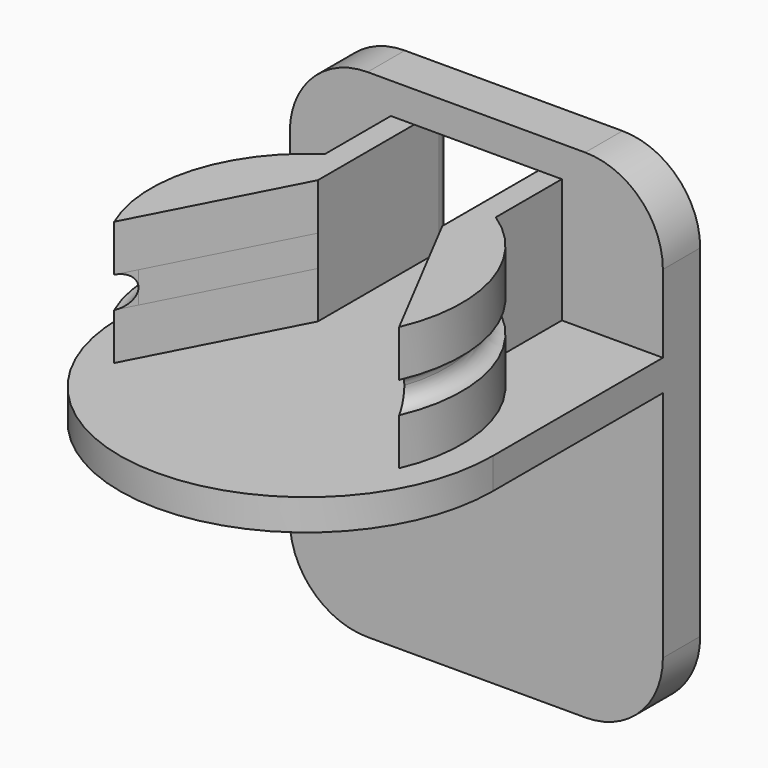
from build123d import *

# Parameters (mm, degrees)
F1_DEPTH     = 2
F3_DEPTH     = 3
F5_DEPTH     = 2
F7_DEPTH     = 3
F8_T4_ANGLE  = 102.3969146675
F8_T10_ANGLE = 102.3969146675
F8_T16_ANGLE = 102.3969146675
F8_T22_ANGLE = 102.3969146675
F8_T26_ANGLE = 121.7069479791
F8_T28_ANGLE = 121.7069479791
F8_T30_ANGLE = 121.7069479791
F8_T32_ANGLE = 121.7069479791
F9_W         = 24
F9_H         = 22.6653645039
F10_DEPTH    = 10
F11_W        = 24
F11_H        = 32
F11_W_2      = 8
F11_H_2      = 8
F12_DEPTH    = 3
F13_R        = 1
F14_R        = 5
F15_W        = 24
F15_H        = 13.6653645039
F16_DEPTH    = 2


# Not quite as in the source:
# - a fillet or chamfer that OpenCascade refuses, or shapes differently, is made with other operations: its cross-section is extruded or revolved along the edge and cut away or added


with BuildPart() as f1:
    # F0 (on Top) → F1 (new body)
    with BuildSketch(Plane.XY):
        with BuildLine():
            ThreePointArc((5.5, 1.5), (0, 24.1653645039), (-5.5, 1.5))
            Line((-5.5, 1.5), (-5.5, -1.5))
            ThreePointArc((-5.5, -1.5), (0, -24.1653645039), (5.5, -1.5))
            Line((5.5, -1.5), (5.5, 1.5))
        make_face()
    extrude(amount=F1_DEPTH)

    # F2 (on face) → F3 (join)
    with BuildSketch(Plane.XY.offset(2)):
        with BuildLine():
            Line((9.7844830762, 19.1125863177), (8.6602540378, 17.1653645039))
            ThreePointArc((8.6602540378, 17.1653645039), (9.4991255677, 9.0402063559), (4, 3.0002131139))
            Line((4, 3.0002131139), (4, -6.2432010007))
            Line((4, -6.2432010007), (9.1651513899, -16.1653645039))
            ThreePointArc((9.1651513899, -16.1653645039), (9.5868378212, -9.3206253964), (5.5, -3.8137179596))
            Line((5.5, -3.8137179596), (5.5, 1.5))
            ThreePointArc((5.5, 1.5), (11.6599594736, 9.3289327537), (9.7844830762, 19.1125863177))
        make_face()
        with BuildLine():
            ThreePointArc((-4, 3.0002131139), (-9.4991255677, 9.0402063559), (-8.6602540378, 17.1653645039))
            Line((-8.6602540378, 17.1653645039), (-9.7844830762, 19.1125863177))
            ThreePointArc((-9.7844830762, 19.1125863177), (-11.6599594736, 9.3289327537), (-5.5, 1.5))
            Line((-5.5, 1.5), (-5.5, -3.8137179596))
            ThreePointArc((-5.5, -3.8137179596), (-9.5868378212, -9.3206253964), (-9.1651513899, -16.1653645039))
            Line((-9.1651513899, -16.1653645039), (-4, -6.2432010007))
            Line((-4, -6.2432010007), (-4, 3.0002131139))
        make_face()
    extrude(amount=F3_DEPTH)

    # F4 (on face) → F5 (join)
    with BuildSketch(Plane.XY.offset(5)):
        with BuildLine():
            Line((-8.0717844057, 16.1461052023), (-9.7844830762, 19.1125863177))
            ThreePointArc((-9.7844830762, 19.1125863177), (-11.6599594736, 9.3289327537), (-5.5, 1.5))
            Line((-5.5, 1.5), (-5.5, -5.0414610795))
            ThreePointArc((-5.5, -5.0414610795), (-8.6043935433, -9.5263473097), (-8.5483759414, -14.980549891))
            Line((-8.5483759414, -14.980549891), (-4, -6.2432010007))
            Line((-4, -6.2432010007), (-4, 4.1031067556))
            ThreePointArc((-4, 4.1031067556), (-8.5258693153, 9.2827350759), (-8.0717844057, 16.1461052023))
        make_face()
        with BuildLine():
            ThreePointArc((5.5, 1.5), (11.6599594736, 9.3289327537), (9.7844830762, 19.1125863177))
            Line((9.7844830762, 19.1125863177), (8.0717844057, 16.1461052023))
            ThreePointArc((8.0717844057, 16.1461052023), (8.5258693153, 9.2827350759), (4, 4.1031067556))
            Line((4, 4.1031067556), (4, -6.2432010007))
            Line((4, -6.2432010007), (8.5483759414, -14.980549891))
            ThreePointArc((8.5483759414, -14.980549891), (8.6043935433, -9.5263473097), (5.5, -5.0414610795))
            Line((5.5, -5.0414610795), (5.5, 1.5))
        make_face()
    extrude(amount=F5_DEPTH)

    # F6 (on face) → F7 (join)
    with BuildSketch(Plane.XY.offset(7)):
        with BuildLine():
            Line((9.7844830762, 19.1125863177), (8.6602540378, 17.1653645039))
            ThreePointArc((8.6602540378, 17.1653645039), (9.4991255677, 9.0402063559), (4, 3.0002131139))
            Line((4, 3.0002131139), (4, -6.2432010007))
            Line((4, -6.2432010007), (9.1651513899, -16.1653645039))
            ThreePointArc((9.1651513899, -16.1653645039), (9.5868378212, -9.3206253964), (5.5, -3.8137179596))
            Line((5.5, -3.8137179596), (5.5, 1.5))
            ThreePointArc((5.5, 1.5), (11.6599594736, 9.3289327537), (9.7844830762, 19.1125863177))
        make_face()
        with BuildLine():
            ThreePointArc((-4, 3.0002131139), (-9.4991255677, 9.0402063559), (-8.6602540378, 17.1653645039))
            Line((-8.6602540378, 17.1653645039), (-9.7844830762, 19.1125863177))
            ThreePointArc((-9.7844830762, 19.1125863177), (-11.6599594736, 9.3289327537), (-5.5, 1.5))
            Line((-5.5, 1.5), (-5.5, -3.8137179596))
            ThreePointArc((-5.5, -3.8137179596), (-9.5868378212, -9.3206253964), (-9.1651513899, -16.1653645039))
            Line((-9.1651513899, -16.1653645039), (-4, -6.2432010007))
            Line((-4, -6.2432010007), (-4, 3.0002131139))
        make_face()
    extrude(amount=F7_DEPTH)

    # F8: fillet of radius 1 on 8 edges, made by hand


with BuildPart() as f8_tool2:
    # F8_s3 → F8_t4 (revolve)
    with BuildSketch(Plane(origin=(-4.1871135562, -1.6705281924, 0), x_dir=(0, 0, 1), z_dir=(0.9288065548, 0.3705649522, 0))):
        with BuildLine():
            ThreePointArc((6, 2.2992702923), (5.2928932188, 2.0063770734), (5, 1.2992702923))
            Line((5, 1.2992702923), (5, 2.2992702923))
            Line((5, 2.2992702923), (6, 2.2992702923))
        make_face()
    revolve(axis=Axis((0, -12.1653645039, 5), (0, 0, 1)), revolution_arc=F8_T4_ANGLE)

    split(bisect_by=Plane(origin=(-0.5900874414, 0.3071800789, 0), x_dir=(0, 0, 1), z_dir=(-0.8870108332, 0.4617486132, 0)), keep=Keep.TOP)

    split(bisect_by=Plane.YZ.offset(-4), keep=Keep.BOTTOM)


with BuildPart() as f1_1:
    add(f1.part)

    # F8_t1: union F8_tool2
    add(f8_tool2.part)


with BuildPart() as f8_tool8:
    # F8_s9 → F8_t10 (revolve)
    with BuildSketch(Plane(origin=(-4.1871135562, -1.6705281924, 0), x_dir=(0, 0, 1), z_dir=(0.9288065548, 0.3705649522, 0))):
        with BuildLine():
            ThreePointArc((7, 1.2992702923), (6.7071067812, 2.0063770734), (6, 2.2992702923))
            Line((6, 2.2992702923), (7, 2.2992702923))
            Line((7, 2.2992702923), (7, 1.2992702923))
        make_face()
    revolve(axis=Axis((0, -12.1653645039, 7), (0, 0, 1)), revolution_arc=F8_T10_ANGLE)

    split(bisect_by=Plane(origin=(-0.5900874414, 0.3071800789, 0), x_dir=(0, 0, 1), z_dir=(-0.8870108332, 0.4617486132, 0)), keep=Keep.TOP)

    split(bisect_by=Plane.YZ.offset(-4), keep=Keep.BOTTOM)


with BuildPart() as f1_2:
    add(f1_1.part)

    # F8_t7: union F8_tool8
    add(f8_tool8.part)


with BuildPart() as f8_tool14:
    # F8_s15 → F8_t16 (revolve)
    with BuildSketch(Plane(origin=(-5.6514123525, -8.3322514997, 0), x_dir=(0, 0, 1), z_dir=(-0.561323531, -0.8275964557, 0))):
        with BuildLine():
            ThreePointArc((6, -15.828705359), (6.7071067812, -16.1215985778), (7, -16.828705359))
            Line((7, -16.828705359), (7, -15.828705359))
            Line((7, -15.828705359), (6, -15.828705359))
        make_face()
    revolve(axis=Axis((0, -12.1653645039, 7), (0, 0, 1)), revolution_arc=F8_T16_ANGLE)

    split(bisect_by=Plane.YZ.offset(4), keep=Keep.TOP)

    split(bisect_by=Plane(origin=(0.5900874414, 0.3071800789, 0), x_dir=(0, 0, 1), z_dir=(0.8870108332, 0.4617486132, 0)), keep=Keep.TOP)


with BuildPart() as f1_3:
    add(f1_2.part)

    # F8_t13: union F8_tool14
    add(f8_tool14.part)


with BuildPart() as f8_tool20:
    # F8_s21 → F8_t22 (revolve)
    with BuildSketch(Plane(origin=(-5.6514123525, -8.3322514997, 0), x_dir=(0, 0, 1), z_dir=(-0.561323531, -0.8275964557, 0))):
        with BuildLine():
            ThreePointArc((5, -16.828705359), (5.2928932188, -16.1215985778), (6, -15.828705359))
            Line((6, -15.828705359), (5, -15.828705359))
            Line((5, -15.828705359), (5, -16.828705359))
        make_face()
    revolve(axis=Axis((0, -12.1653645039, 5), (0, 0, 1)), revolution_arc=F8_T22_ANGLE)

    split(bisect_by=Plane.YZ.offset(4), keep=Keep.TOP)

    split(bisect_by=Plane(origin=(0.5900874414, 0.3071800789, 0), x_dir=(0, 0, 1), z_dir=(0.8870108332, 0.4617486132, 0)), keep=Keep.TOP)


with BuildPart() as f1_4:
    add(f1_3.part)

    # F8_t19: union F8_tool20
    add(f8_tool20.part)

    # F8_s25 → F8_t26 (revolve, cut)
    with BuildSketch(Plane(origin=(-6.0530874143, 6.6819786169, 0), x_dir=(0, 0, 1), z_dir=(-0.6713698624, 0.7411224648, 0))):
        with BuildLine():
            ThreePointArc((7, 18.1674590926), (6.7071067812, 17.4603523114), (6, 17.1674590926))
            Line((6, 17.1674590926), (7, 17.1674590926))
            Line((7, 17.1674590926), (7, 18.1674590926))
        make_face()
    revolve(axis=Axis((0, 12.1653645039, 7), (0, 0, -1)), revolution_arc=F8_T26_ANGLE, mode=Mode.SUBTRACT)

    # F8_s27 → F8_t28 (revolve, cut)
    with BuildSketch(Plane(origin=(-2.1730837017, 0.4014208952, 0), x_dir=(0, 0, 1), z_dir=(0.9833630917, -0.1816508459, 0))):
        with BuildLine():
            ThreePointArc((6, -2.9629704506), (6.7071067812, -2.6700772318), (7, -1.9629704506))
            Line((7, -1.9629704506), (7, -2.9629704506))
            Line((7, -2.9629704506), (6, -2.9629704506))
        make_face()
    revolve(axis=Axis((0, 12.1653645039, 7), (0, 0, -1)), revolution_arc=F8_T28_ANGLE, mode=Mode.SUBTRACT)

    # F8_s29 → F8_t30 (revolve, cut)
    with BuildSketch(Plane(origin=(-2.1730837017, 0.4014208952, 0), x_dir=(0, 0, 1), z_dir=(0.9833630917, -0.1816508459, 0))):
        with BuildLine():
            ThreePointArc((5, -1.9629704506), (5.2928932188, -2.6700772318), (6, -2.9629704506))
            Line((6, -2.9629704506), (5, -2.9629704506))
            Line((5, -2.9629704506), (5, -1.9629704506))
        make_face()
    revolve(axis=Axis((0, 12.1653645039, 5), (0, 0, -1)), revolution_arc=F8_T30_ANGLE, mode=Mode.SUBTRACT)

    # F8_s31 → F8_t32 (revolve, cut)
    with BuildSketch(Plane(origin=(-6.0530874143, 6.6819786169, 0), x_dir=(0, 0, 1), z_dir=(-0.6713698624, 0.7411224648, 0))):
        with BuildLine():
            ThreePointArc((6, 17.1674590926), (5.2928932188, 17.4603523114), (5, 18.1674590926))
            Line((5, 18.1674590926), (5, 17.1674590926))
            Line((5, 17.1674590926), (6, 17.1674590926))
        make_face()
    revolve(axis=Axis((0, 12.1653645039, 5), (0, 0, -1)), revolution_arc=F8_T32_ANGLE, mode=Mode.SUBTRACT)

    # F9 (on face) → F10 (cut)
    with BuildSketch(Plane.XY.offset(10)):
        with Locations((0, 12.8326822519)):
            Rectangle(F9_W, F9_H)
    extrude(amount=-F10_DEPTH, mode=Mode.SUBTRACT)

    # F11 (on face) → F12 (join)
    with BuildSketch(Plane(origin=(0, 1.5, 0), x_dir=(-1, 0, 0), z_dir=(0, 1, 0))):
        with Locations((0, -4)):
            Rectangle(F11_W, F11_H)
        with Locations((0, 6)):
            Rectangle(F11_W_2, F11_H_2, mode=Mode.SUBTRACT)
    extrude(amount=F12_DEPTH)

    # F13
    f13_edges = [f1_4.edges().sort_by_distance(p)[0] for p in [
        (0, 4.5, 10),
        (4, 4.5, 6),
        (-4, 4.5, 6),
        (0, 4.5, 2),
    ]]
    fillet(f13_edges, radius=F13_R)

    # F14
    f14_edges = [f1_4.edges().sort_by_distance(p)[0] for p in [
        (12, 3, 12),
        (-12, 3, 12),
        (-12, 3, -20),
        (12, 3, -20),
    ]]
    fillet(f14_edges, radius=F14_R)

    # F15 (on face) → F16 (join)
    with BuildSketch(Plane(origin=(0, 0, 0), x_dir=(1, 0, 0), z_dir=(0, 0, -1))):
        with Locations((0, 5.3326822519)):
            Rectangle(F15_W, F15_H)
    extrude(amount=-F16_DEPTH)


solid = f1_4.part
